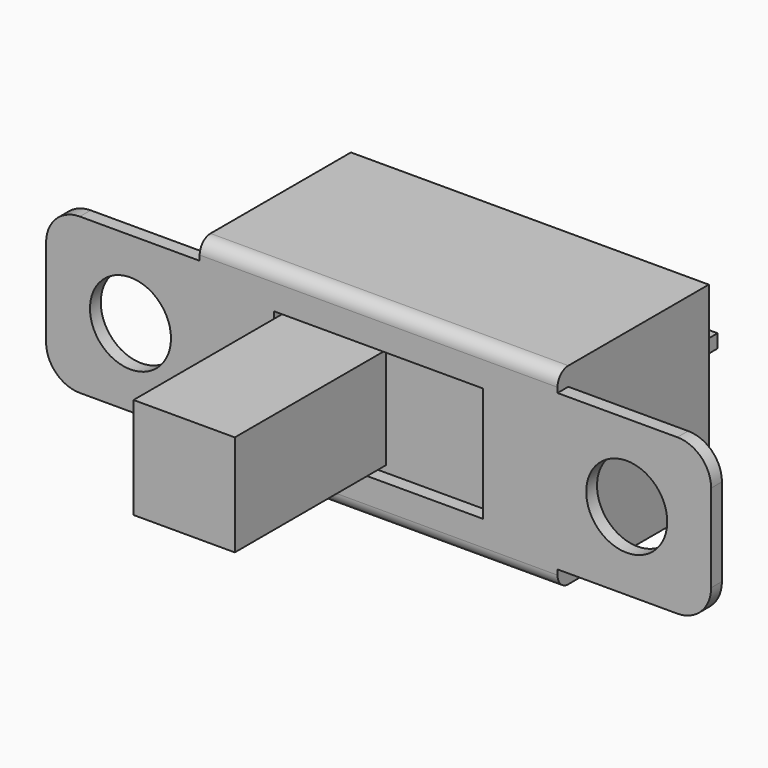
from build123d import *

# Parameters (mm, degrees)
F0_W      = 4.55
F0_H      = 4.6
F0_W_2    = 10.6
F0_H_2    = 0.55
F1_DEPTH  = 0.4
F2_R      = 1.2
F3_DEPTH  = 0.5
F4_R      = 0.39999
F5_W      = 10.6
F5_H      = 5.7
F6_DEPTH  = 5.2
F7_R      = 1
F8_W      = 6.2
F8_H      = 3.4
F9_DEPTH  = 0.4
F10_W     = 3
F10_H     = 3
F11_DEPTH = 5.6
F12_W     = 7.6
F12_H     = 0.4
F13_DEPTH = 2.2


# Not quite as in the source:
# - a fillet or chamfer is up to 0.001 mm smaller than in the source, because OpenCascade refuses the exact size


with BuildPart() as f1:
    # F0 (on Front) → F1 (new body)
    with BuildSketch(Plane.XZ):
        with Locations((7.575, 0)):
            Rectangle(F0_W, F0_H)
        with Locations((0, -2.575)):
            Rectangle(F0_W_2, F0_H_2)
        Rectangle(F0_W_2, F0_H)
        with Locations((-7.575, 0)):
            Rectangle(F0_W, F0_H)
        with Locations((0, 2.575)):
            Rectangle(F0_W_2, F0_H_2)
    extrude(amount=F1_DEPTH)

    # F2 (on face) → F3 (cut)
    with BuildSketch(Plane.XZ.offset(0.4)):
        with Locations((-7.35, 0)):
            Circle(F2_R)
        with Locations((7.35, 0)):
            Circle(F2_R)
    extrude(amount=-F3_DEPTH, mode=Mode.SUBTRACT)

    # F4 (radius 0.4 in the source; OpenCascade refuses exactly that, so slightly less here)
    f4_edges = [f1.edges().sort_by_distance(p)[0] for p in [
        (0, -0.4, 2.85),
        (0, -0.4, -2.85),
    ]]
    fillet(f4_edges, radius=F4_R)

    # F5 (on face) → F6 (join)
    with BuildSketch(Plane(origin=(0, 0, 0), x_dir=(-1, 0, 0), z_dir=(0, 1, 0))):
        Rectangle(F5_W, F5_H)
    extrude(amount=F6_DEPTH)

    # F7
    f7_edges = [f1.edges().sort_by_distance(p)[0] for p in [
        (9.85, -0.2, 2.3),
        (9.85, -0.2, -2.3),
        (-9.85, -0.2, -2.3),
        (-9.85, -0.2, 2.3),
    ]]
    fillet(f7_edges, radius=F7_R)

    # F8 (on face) → F9 (cut)
    with BuildSketch(Plane.XZ.offset(0.4)):
        Rectangle(F8_W, F8_H)
    extrude(amount=-F9_DEPTH, mode=Mode.SUBTRACT)

    # F10 (on face) → F11 (join)
    with BuildSketch(Plane.XZ):
        with Locations((-1.6, 0)):
            Rectangle(F10_W, F10_H)
    extrude(amount=F11_DEPTH)

    # F12 (on face) → F13 (join)
    with BuildSketch(Plane(origin=(0, 5.2, 0), x_dir=(-1, 0, 0), z_dir=(0, 1, 0))):
        Rectangle(F12_W, F12_H)
    extrude(amount=F13_DEPTH)


solid = f1.part
